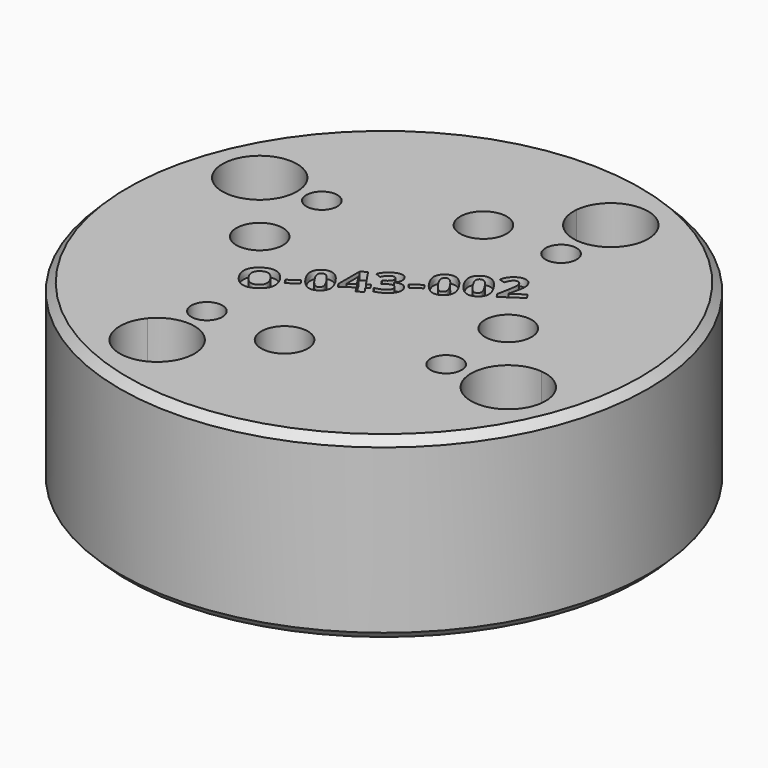
from build123d import *

# Parameters (mm, degrees)
F0_R         = 34
F0_R_2       = 2
F0_R_3       = 3
F1_DEPTH     = 23
F2_TEXT_SIZE = 6.1259651586
F3_DEPTH     = 1
F4_SIZE      = 1


# Not quite as in the source:
# - a feature names something its author has since deleted; it is built from what else it names
# - Text() gives the source's letters only with a copy of the font that has no kerning and outlines rounded to 1/6400 em; it was checked with that copy


with BuildPart() as f1:
    # F0 (on Top) → F1 (new body)
    with BuildSketch(Plane.XY):
        Circle(F0_R)
        with BuildLine():
            ThreePointArc((13.6837118225, 20.922620074), (21.9896884421, 11.8934268493), (25, 0))
            ThreePointArc((25, 0), (24.8618032514, -2.6250217314), (24.4487408728, -5.2210219054))
            ThreePointArc((24.4487408728, -5.2210219054), (27.5492221816, -6.7684335214), (28.8, -10))
            ThreePointArc((28.8, -10), (26.0332949067, -14.3480698962), (20.922620074, -13.6837118225))
            ThreePointArc((20.922620074, -13.6837118225), (9.5187451314, -23.1169524619), (-5.2210219054, -24.4487408728))
            ThreePointArc((-5.2210219054, -24.4487408728), (-11.8461538462, -28.4307692308), (-13.6837118225, -20.922620074))
            ThreePointArc((-13.6837118225, -20.922620074), (-23.1169524619, -9.5187451314), (-24.4487408728, 5.2210219054))
            ThreePointArc((-24.4487408728, 5.2210219054), (-28.4307692308, 11.8461538462), (-20.922620074, 13.6837118225))
            ThreePointArc((-20.922620074, 13.6837118225), (-9.5187451314, 23.1169524619), (5.2210219054, 24.4487408728))
            ThreePointArc((5.2210219054, 24.4487408728), (10.2246165017, 28.7947416434), (14.8, 24))
            ThreePointArc((14.8, 24), (14.5123063254, 22.363206908), (13.6837118225, 20.922620074))
        make_face(mode=Mode.SUBTRACT)
        with BuildLine():
            ThreePointArc((24.4487408728, -5.2210219054), (24.8618032514, -2.6250217314), (25, 0))
            ThreePointArc((25, 0), (21.9896884421, 11.8934268493), (13.6837118225, 20.922620074))
            ThreePointArc((13.6837118225, 20.922620074), (8.1538461538, 19.5692307692), (5.2210219054, 24.4487408728))
            ThreePointArc((5.2210219054, 24.4487408728), (-9.5187451314, 23.1169524619), (-20.922620074, 13.6837118225))
            ThreePointArc((-20.922620074, 13.6837118225), (-19.6519301038, 12.0332949067), (-19.2, 10))
            ThreePointArc((-19.2, 10), (-20.7684335214, 6.4507778184), (-24.4487408728, 5.2210219054))
            ThreePointArc((-24.4487408728, 5.2210219054), (-23.1169524619, -9.5187451314), (-13.6837118225, -20.922620074))
            ThreePointArc((-13.6837118225, -20.922620074), (-8.363206908, -19.4876936746), (-5.2, -24))
            ThreePointArc((-5.2, -24), (-5.2052583566, -24.2246165017), (-5.2210219054, -24.4487408728))
            ThreePointArc((-5.2210219054, -24.4487408728), (9.5187451314, -23.1169524619), (20.922620074, -13.6837118225))
            ThreePointArc((20.922620074, -13.6837118225), (19.5692307692, -8.1538461538), (24.4487408728, -5.2210219054))
        make_face()
        with Locations((-10, -16)):
            Circle(F0_R_2, mode=Mode.SUBTRACT)
        with Locations((0, -16)):
            Circle(F0_R_3, mode=Mode.SUBTRACT)
        with Locations((16, -10)):
            Circle(F0_R_2, mode=Mode.SUBTRACT)
        with Locations((-16, 0)):
            Circle(F0_R_3, mode=Mode.SUBTRACT)
        with Locations((-16, 10)):
            Circle(F0_R_2, mode=Mode.SUBTRACT)
        with Locations((16, 0)):
            Circle(F0_R_3, mode=Mode.SUBTRACT)
        with Locations((0, 16)):
            Circle(F0_R_3, mode=Mode.SUBTRACT)
        with Locations((10, 16)):
            Circle(F0_R_2, mode=Mode.SUBTRACT)
    extrude(amount=F1_DEPTH)

    # F2 (on face) → F3 (cut)
    with BuildSketch(Plane.XY.offset(23)):
        with Locations(Location((-11.2023489406, -10.2162094545), (0, 0, 34))):
            Text('O-043-002', F2_TEXT_SIZE, font='Open Sans', font_style=FontStyle.BOLD, text_align=(TextAlign.LEFT, TextAlign.BOTTOM))
    extrude(amount=-F3_DEPTH, mode=Mode.SUBTRACT)

    # F4
    f4_edges = [f1.edges().sort_by_distance(p)[0] for p in [
        (-34, 0, 23),
        (-34, 0, 0),
    ]]
    chamfer(f4_edges, length=F4_SIZE)


solid = f1.part
